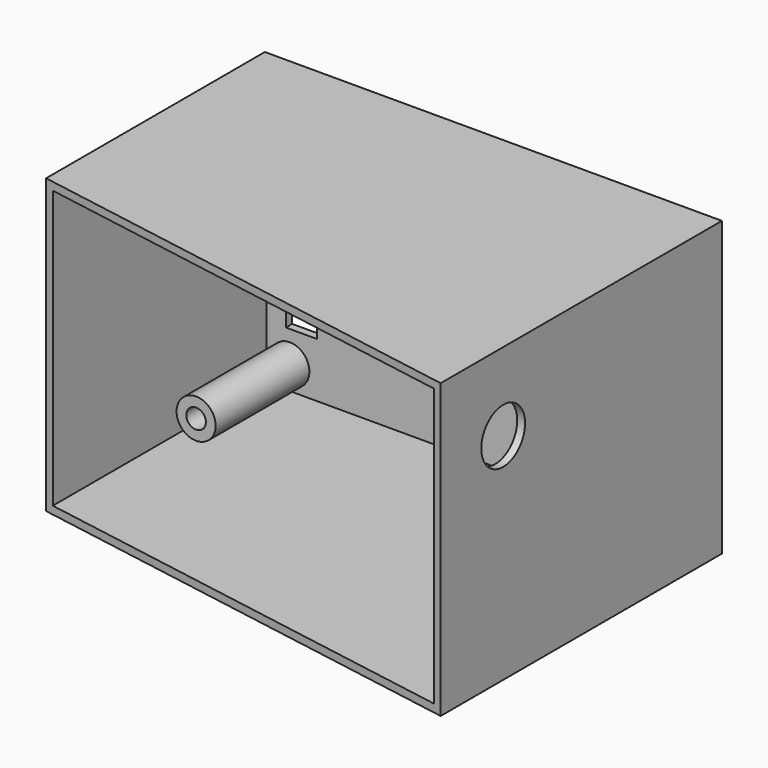
from build123d import *

# Parameters (mm, degrees)
F0_W     = 58.5
F0_H     = 37.5
F0_W_2   = 4
F0_H_2   = 15
F1_DEPTH = 45
F2_T     = -1
F4_DEPTH = 52.9
F5_R     = 3.5
F6_DEPTH = 25
F7_DEPTH = 25
F8_R     = 2.5
F8_R_2   = 1.25
F9_DEPTH = 15


# Not quite as in the source:
# - a feature names something its author has since deleted; it is built from what else it names


with BuildPart() as f1:
    # F0 (on Front) → F1 (new body)
    with BuildSketch(Plane.XZ):
        with Locations((-135.4310402274, -41.6724174619)):
            Rectangle(F0_W, F0_H)
        with Locations((-159.1810402274, -44.9224174619)):
            Rectangle(F0_W_2, F0_H_2, mode=Mode.SUBTRACT)
        with Locations((-159.1810402274, -44.9224174619)):
            Rectangle(F0_W_2, F0_H_2)
    extrude(amount=F1_DEPTH)

    # F2
    f2_openings = [f1.faces().sort_by_distance(p)[0] for p in [
        (-135.43104, -45, -41.672417),
    ]]
    offset(amount=F2_T, openings=f2_openings)

    # F3 (on face) → F4 (cut)
    with BuildSketch(Plane(origin=(0, 0, -60.4224174619), x_dir=(1, 0, 0), z_dir=(0, 0, -1))):
        Polygon((-164.6810402274, 45), (-164.6810402274, 35), (-106.1810402274, 45), align=None)
    extrude(amount=-F4_DEPTH, mode=Mode.SUBTRACT)

    # F5 (on face) → F6 (cut)
    with BuildSketch(Plane.YZ.offset(-106.1810402274)):
        with Locations((-35, -32.9224174619)):
            Circle(F5_R)
    extrude(amount=-F6_DEPTH, mode=Mode.SUBTRACT)

    # F0 (on Front) → F7 (cut)
    with BuildSketch(Plane.XZ):
        with Locations((-159.1810402274, -44.9224174619)):
            Rectangle(F0_W_2, F0_H_2)
    extrude(amount=F7_DEPTH, mode=Mode.SUBTRACT)

    # F8 (on face) → F9 (join)
    with BuildSketch(Plane.XZ.offset(1)):
        with Locations((-110.1810402274, -26.9224174619)):
            Circle(F8_R)
        with Locations((-110.1810402274, -26.9224174619)):
            Circle(F8_R_2, mode=Mode.SUBTRACT)
        with Locations((-110.1810402274, -56.4224174619)):
            Circle(F8_R)
        with Locations((-110.1810402274, -56.4224174619)):
            Circle(F8_R_2, mode=Mode.SUBTRACT)
        with Locations((-160.6810402274, -56.4224174619)):
            Circle(F8_R)
        with Locations((-160.6810402274, -56.4224174619)):
            Circle(F8_R_2, mode=Mode.SUBTRACT)
        with Locations((-160.6810402274, -26.9224174619)):
            Circle(F8_R)
        with Locations((-160.6810402274, -26.9224174619)):
            Circle(F8_R_2, mode=Mode.SUBTRACT)
    extrude(amount=F9_DEPTH)


solid = f1.part
